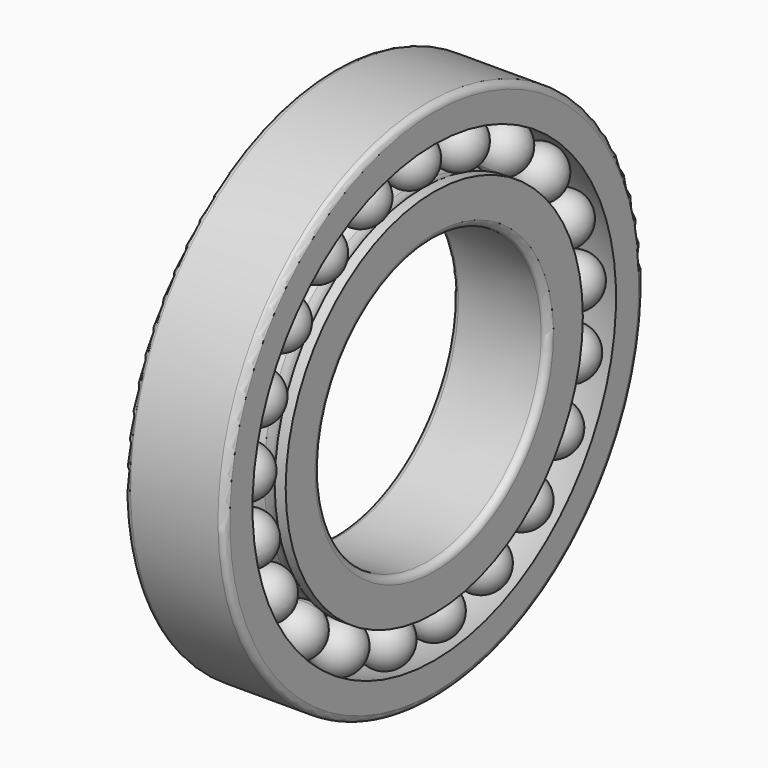
from build123d import *

# Parameters (mm, degrees)
F4_COUNT = 21


with BuildPart() as f1:
    # F0 (on Front) → F1 (revolve)
    with BuildSketch(Plane.XZ):
        with BuildLine():
            ThreePointArc((-11.5, 52), (0, 53.4849147412), (11.5, 52))
            Line((11.5, 52), (11.5, 58.5))
            ThreePointArc((11.5, 58.5), (11.0606601718, 59.5606601718), (10, 60))
            Line((10, 60), (-10, 60))
            ThreePointArc((-10, 60), (-11.0606601718, 59.5606601718), (-11.5, 58.5))
            Line((-11.5, 58.5), (-11.5, 52))
        make_face()
    revolve(axis=Axis((5.75, 0, 0), (1, 0, 0)))


with BuildPart() as f1b:
    # F0 (on Front) → F1, piece 2 (revolve)
    with BuildSketch(Plane.XZ):
        with BuildLine():
            ThreePointArc((-11.5, 35.428810631), (-11.0951838715, 34.4038363447), (-10.0992369499, 33.9320968883))
            Line((-10.0992369499, 33.9320968883), (9.9007630501, 32.6060323639))
            ThreePointArc((9.9007630501, 32.6060323639), (11.0249742863, 33.0075622352), (11.5, 34.1027461067))
            Line((11.5, 34.1027461067), (11.5, 42.4999977946))
            Line((11.5, 42.4999977946), (8.9903687328, 42.4999977946))
            ThreePointArc((8.9903687328, 42.4999977946), (7.4455815609, 41.7556833649), (5.75, 41.4999988973))
            ThreePointArc((5.75, 41.4999988973), (4.0544184391, 41.7556833649), (2.5096312672, 42.4999977946))
            Line((2.5096312672, 42.4999977946), (-2.5096312672, 42.4999977946))
            ThreePointArc((-2.5096312672, 42.4999977946), (-4.0544184391, 41.7556833649), (-5.75, 41.4999988973))
            ThreePointArc((-5.75, 41.4999988973), (-7.4455815609, 41.7556833649), (-8.9903687328, 42.4999977946))
            Line((-8.9903687328, 42.4999977946), (-11.5, 42.4999977946))
            Line((-11.5, 42.4999977946), (-11.5, 35.428810631))
        make_face()
    revolve(axis=Axis((5.75, 0, 0), (1, 0, 0)))


with BuildPart() as f2:
    # F0 (on Front) → F2 (revolve)
    with BuildSketch(Plane.XZ):
        with BuildLine():
            Line((-5.75, 47.2499988973), (-5.75, 41.4999988973))
            ThreePointArc((-5.75, 41.4999988973), (-4.0544184391, 41.7556833649), (-2.5096312672, 42.4999977946))
            ThreePointArc((-2.5096312672, 42.4999977946), (-0.2556844675, 48.9455804582), (-5.75, 52.9999988973))
            Line((-5.75, 52.9999988973), (-5.75, 52))
            Line((-5.75, 52), (-5.75, 47.2499988973))
        make_face()
    revolve(axis=Axis((-5.75, 0, 49.6249994487), (0, 0, -1)))


with BuildPart() as f3:
    # F0 (on Front) → F3 (revolve)
    with BuildSketch(Plane.XZ):
        with BuildLine():
            ThreePointArc((5.75, 41.4999988973), (7.4455815609, 41.7556833649), (8.9903687328, 42.4999977946))
            ThreePointArc((8.9903687328, 42.4999977946), (11.2443155325, 48.9455804582), (5.75, 52.9999988973))
            Line((5.75, 52.9999988973), (5.75, 41.4999988973))
        make_face()
    revolve(axis=Axis((5.75, 0, 47.2499988973), (0, 0, -1)))


with BuildPart() as f4_1:
    # F4: instance of F2
    add(f2.part.rotate(Axis((5.75, 0, 0), (1, 0, 0)), 1 * 360 / F4_COUNT))


with BuildPart() as f4_2:
    # F4: instance of F2
    add(f2.part.rotate(Axis((5.75, 0, 0), (1, 0, 0)), 2 * 360 / F4_COUNT))


with BuildPart() as f4_3:
    # F4: instance of F2
    add(f2.part.rotate(Axis((5.75, 0, 0), (1, 0, 0)), 3 * 360 / F4_COUNT))


with BuildPart() as f4_4:
    # F4: instance of F2
    add(f2.part.rotate(Axis((5.75, 0, 0), (1, 0, 0)), 4 * 360 / F4_COUNT))


with BuildPart() as f4_5:
    # F4: instance of F2
    add(f2.part.rotate(Axis((5.75, 0, 0), (1, 0, 0)), 5 * 360 / F4_COUNT))


with BuildPart() as f4_6:
    # F4: instance of F2
    add(f2.part.rotate(Axis((5.75, 0, 0), (1, 0, 0)), 6 * 360 / F4_COUNT))


with BuildPart() as f4_7:
    # F4: instance of F2
    add(f2.part.rotate(Axis((5.75, 0, 0), (1, 0, 0)), 7 * 360 / F4_COUNT))


with BuildPart() as f4_8:
    # F4: instance of F2
    add(f2.part.rotate(Axis((5.75, 0, 0), (1, 0, 0)), 8 * 360 / F4_COUNT))


with BuildPart() as f4_9:
    # F4: instance of F2
    add(f2.part.rotate(Axis((5.75, 0, 0), (1, 0, 0)), 9 * 360 / F4_COUNT))


with BuildPart() as f4_10:
    # F4: instance of F2
    add(f2.part.rotate(Axis((5.75, 0, 0), (1, 0, 0)), 10 * 360 / F4_COUNT))


with BuildPart() as f4_11:
    # F4: instance of F2
    add(f2.part.rotate(Axis((5.75, 0, 0), (1, 0, 0)), 11 * 360 / F4_COUNT))


with BuildPart() as f4_12:
    # F4: instance of F2
    add(f2.part.rotate(Axis((5.75, 0, 0), (1, 0, 0)), 12 * 360 / F4_COUNT))


with BuildPart() as f4_13:
    # F4: instance of F2
    add(f2.part.rotate(Axis((5.75, 0, 0), (1, 0, 0)), 13 * 360 / F4_COUNT))


with BuildPart() as f4_14:
    # F4: instance of F2
    add(f2.part.rotate(Axis((5.75, 0, 0), (1, 0, 0)), 14 * 360 / F4_COUNT))


with BuildPart() as f4_15:
    # F4: instance of F2
    add(f2.part.rotate(Axis((5.75, 0, 0), (1, 0, 0)), 15 * 360 / F4_COUNT))


with BuildPart() as f4_16:
    # F4: instance of F2
    add(f2.part.rotate(Axis((5.75, 0, 0), (1, 0, 0)), 16 * 360 / F4_COUNT))


with BuildPart() as f4_17:
    # F4: instance of F2
    add(f2.part.rotate(Axis((5.75, 0, 0), (1, 0, 0)), 17 * 360 / F4_COUNT))


with BuildPart() as f4_18:
    # F4: instance of F2
    add(f2.part.rotate(Axis((5.75, 0, 0), (1, 0, 0)), 18 * 360 / F4_COUNT))


with BuildPart() as f4_19:
    # F4: instance of F2
    add(f2.part.rotate(Axis((5.75, 0, 0), (1, 0, 0)), 19 * 360 / F4_COUNT))


with BuildPart() as f4_20:
    # F4: instance of F2
    add(f2.part.rotate(Axis((5.75, 0, 0), (1, 0, 0)), 20 * 360 / F4_COUNT))


with BuildPart() as f4_21:
    # F4: instance of F3
    add(f3.part.rotate(Axis((5.75, 0, 0), (1, 0, 0)), 1 * 360 / F4_COUNT))


with BuildPart() as f4_22:
    # F4: instance of F3
    add(f3.part.rotate(Axis((5.75, 0, 0), (1, 0, 0)), 2 * 360 / F4_COUNT))


with BuildPart() as f4_23:
    # F4: instance of F3
    add(f3.part.rotate(Axis((5.75, 0, 0), (1, 0, 0)), 3 * 360 / F4_COUNT))


with BuildPart() as f4_24:
    # F4: instance of F3
    add(f3.part.rotate(Axis((5.75, 0, 0), (1, 0, 0)), 4 * 360 / F4_COUNT))


with BuildPart() as f4_25:
    # F4: instance of F3
    add(f3.part.rotate(Axis((5.75, 0, 0), (1, 0, 0)), 5 * 360 / F4_COUNT))


with BuildPart() as f4_26:
    # F4: instance of F3
    add(f3.part.rotate(Axis((5.75, 0, 0), (1, 0, 0)), 6 * 360 / F4_COUNT))


with BuildPart() as f4_27:
    # F4: instance of F3
    add(f3.part.rotate(Axis((5.75, 0, 0), (1, 0, 0)), 7 * 360 / F4_COUNT))


with BuildPart() as f4_28:
    # F4: instance of F3
    add(f3.part.rotate(Axis((5.75, 0, 0), (1, 0, 0)), 8 * 360 / F4_COUNT))


with BuildPart() as f4_29:
    # F4: instance of F3
    add(f3.part.rotate(Axis((5.75, 0, 0), (1, 0, 0)), 9 * 360 / F4_COUNT))


with BuildPart() as f4_30:
    # F4: instance of F3
    add(f3.part.rotate(Axis((5.75, 0, 0), (1, 0, 0)), 10 * 360 / F4_COUNT))


with BuildPart() as f4_31:
    # F4: instance of F3
    add(f3.part.rotate(Axis((5.75, 0, 0), (1, 0, 0)), 11 * 360 / F4_COUNT))


with BuildPart() as f4_32:
    # F4: instance of F3
    add(f3.part.rotate(Axis((5.75, 0, 0), (1, 0, 0)), 12 * 360 / F4_COUNT))


with BuildPart() as f4_33:
    # F4: instance of F3
    add(f3.part.rotate(Axis((5.75, 0, 0), (1, 0, 0)), 13 * 360 / F4_COUNT))


with BuildPart() as f4_34:
    # F4: instance of F3
    add(f3.part.rotate(Axis((5.75, 0, 0), (1, 0, 0)), 14 * 360 / F4_COUNT))


with BuildPart() as f4_35:
    # F4: instance of F3
    add(f3.part.rotate(Axis((5.75, 0, 0), (1, 0, 0)), 15 * 360 / F4_COUNT))


with BuildPart() as f4_36:
    # F4: instance of F3
    add(f3.part.rotate(Axis((5.75, 0, 0), (1, 0, 0)), 16 * 360 / F4_COUNT))


with BuildPart() as f4_37:
    # F4: instance of F3
    add(f3.part.rotate(Axis((5.75, 0, 0), (1, 0, 0)), 17 * 360 / F4_COUNT))


with BuildPart() as f4_38:
    # F4: instance of F3
    add(f3.part.rotate(Axis((5.75, 0, 0), (1, 0, 0)), 18 * 360 / F4_COUNT))


with BuildPart() as f4_39:
    # F4: instance of F3
    add(f3.part.rotate(Axis((5.75, 0, 0), (1, 0, 0)), 19 * 360 / F4_COUNT))


with BuildPart() as f4_40:
    # F4: instance of F3
    add(f3.part.rotate(Axis((5.75, 0, 0), (1, 0, 0)), 20 * 360 / F4_COUNT))


solid = Compound([f1.part, f1b.part, f2.part, f3.part, f4_1.part, f4_2.part, f4_3.part, f4_4.part, f4_5.part, f4_6.part, f4_7.part, f4_8.part, f4_9.part, f4_10.part, f4_11.part, f4_12.part, f4_13.part, f4_14.part, f4_15.part, f4_16.part, f4_17.part, f4_18.part, f4_19.part, f4_20.part, f4_21.part, f4_22.part, f4_23.part, f4_24.part, f4_25.part, f4_26.part, f4_27.part, f4_28.part, f4_29.part, f4_30.part, f4_31.part, f4_32.part, f4_33.part, f4_34.part, f4_35.part, f4_36.part, f4_37.part, f4_38.part, f4_39.part, f4_40.part])
